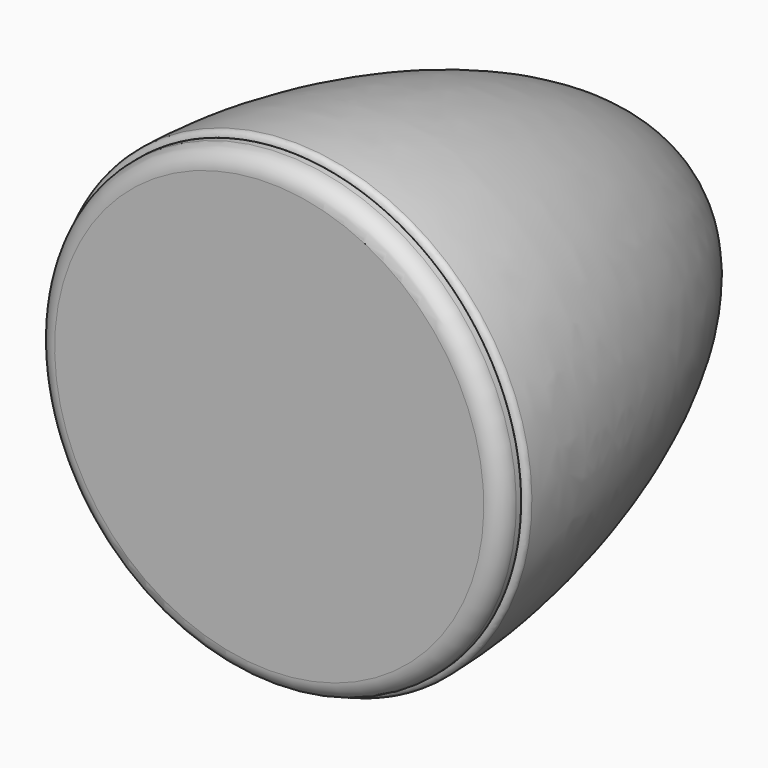
from build123d import *

# Parameters (mm, degrees)
F2_R = 0.3
F3_R = 0.099


# Not quite as in the source:
# - a fillet or chamfer is up to 0.001 mm smaller than in the source, because OpenCascade refuses the exact size


with BuildPart() as f1:
    # F0 (on Right) → F1 (revolve)
    with BuildSketch(Plane.YZ):
        with BuildLine():
            Line((0, -3.8685), (0, -3.9685))
            add(Edge.make_bspline(
                [(0, -3.9685), (2.8934291891, -3.9685), (7.72, -2.4295626208), (7.72, 0)],
                knots=[0, 0, 0, 0, 8.6802875672, 8.6802875672, 8.6802875672, 8.6802875672], degree=3))
            Line((7.72, 0), (-0.4, 0))
            Line((-0.4, 0), (-0.4, -3.8685))
            Line((-0.4, -3.8685), (0, -3.8685))
        make_face()
    revolve(axis=Axis((0, 0.1287413618, 0), (0, 1, 0)))

    # F2
    f2_edges = [f1.edges().sort_by_distance(p)[0] for p in [
        (0, -0.4, 3.8685),
    ]]
    fillet(f2_edges, radius=F2_R)

    # F3 (radius 0.1 in the source; OpenCascade refuses exactly that, so slightly less here)
    f3_edges = [f1.edges().sort_by_distance(p)[0] for p in [
        (0, 0, 3.9685),
    ]]
    fillet(f3_edges, radius=F3_R)


solid = f1.part
